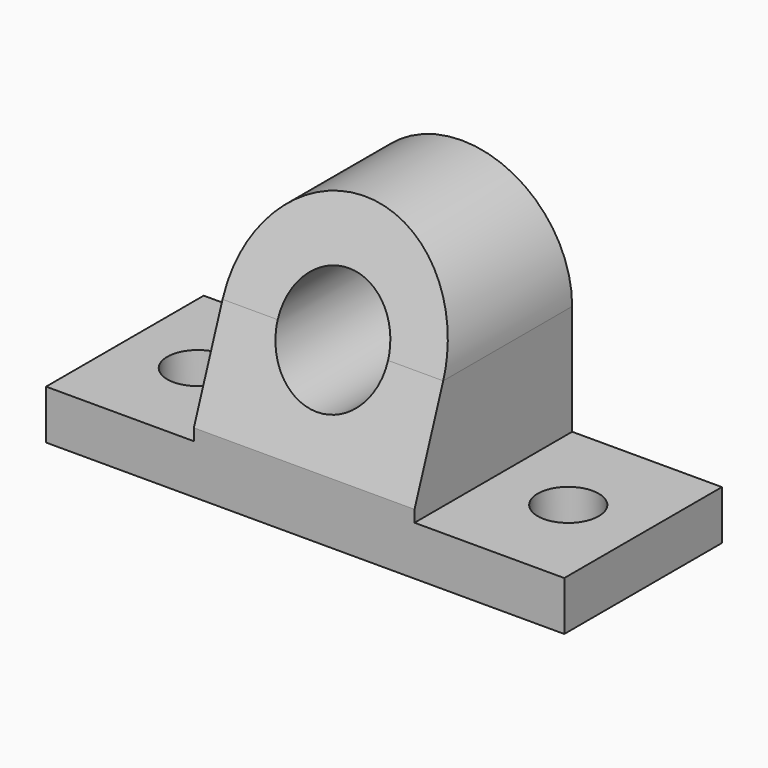
from build123d import *

# Parameters (mm, degrees)
F0_R     = 14.224
F1_DEPTH = 50.8
F2_R     = 7.874
F3_DEPTH = 25.4
F5_DEPTH = 76.2


# Not quite as in the source:
# - a feature names something its author has since deleted; it is built from what else it names


with BuildPart() as f1:
    # F0 (on Front) → F1 (new body)
    with BuildSketch(Plane.XZ):
        with BuildLine():
            Line((28.448, 0), (28.448, 28.448))
            ThreePointArc((28.448, 28.448), (0, 56.896), (-28.448, 28.448))
            Line((-28.448, 28.448), (-28.448, 0))
            Line((-28.448, 0), (-66.548, 0))
            Line((-66.548, 0), (-66.548, -12.7))
            Line((-66.548, -12.7), (67.056, -12.7))
            Line((67.056, -12.7), (67.056, 0))
            Line((67.056, 0), (28.448, 0))
        make_face()
        with Locations((0, 28.448)):
            Circle(F0_R, mode=Mode.SUBTRACT)
    extrude(amount=F1_DEPTH)

    # F2 (on face) → F3 (cut)
    with BuildSketch(Plane.XY):
        with Locations((-47.752, -25.4)):
            Circle(F2_R)
        with Locations((47.752, -25.4)):
            Circle(F2_R)
    extrude(amount=-F3_DEPTH, mode=Mode.SUBTRACT)

    # F4 (on face) → F5 (cut)
    with BuildSketch(Plane.YZ.offset(28.448)):
        Polygon((-50.8, 28.448), (-50.8, 3.048), (-41.5551560496, 28.448), align=None)
        Polygon((-50.8, 28.448), (-41.5551560496, 28.448), (-26.8481459022, 68.8551782879), (-50.8, 64.0367791057), align=None)
    extrude(amount=-F5_DEPTH, mode=Mode.SUBTRACT)


solid = f1.part
